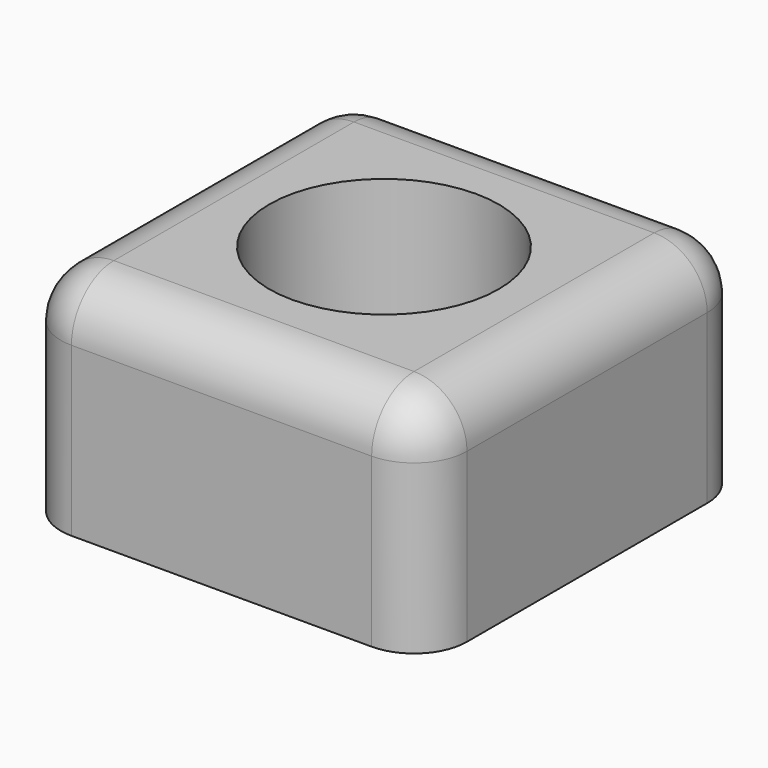
from build123d import *

# Parameters (mm, degrees)
F0_W         = 46
F0_H         = 46
F1_DEPTH     = 25
F3_DEPTH     = 15
F4_R         = 6
F5_T1_DEPTH  = 34
F5_S5_W      = 6
F5_S5_H      = 6
F5_T6_DEPTH  = 6
F5_S11_W     = 6
F5_S11_H     = 6
F5_T12_DEPTH = 6
F5_S17_W     = 6
F5_S17_H     = 6
F5_T18_DEPTH = 6
F5_S23_W     = 6
F5_S23_H     = 6
F5_T24_DEPTH = 6


# Not quite as in the source:
# - a fillet or chamfer that OpenCascade refuses, or shapes differently, is made with other operations: its cross-section is extruded or revolved along the edge and cut away or added


with BuildPart() as f1:
    # F0 (on Top) → F1 (new body)
    with BuildSketch(Plane.XY):
        with Locations((-23, 23)):
            Rectangle(F0_W, F0_H)
    extrude(amount=F1_DEPTH)

    # F2 (on face) → F3 (cut)
    with BuildSketch(Plane.XY.offset(25)):
        with BuildLine():
            ThreePointArc((-10, 23), (-32.1923881554, 32.1923881554), (-23, 10))
            ThreePointArc((-23, 10), (-13.8076118446, 13.8076118446), (-10, 23))
        make_face()
    extrude(amount=-F3_DEPTH, mode=Mode.SUBTRACT)

    # F4
    f4_edges = [f1.edges().sort_by_distance(p)[0] for p in [
        (-23, 0, 25),
        (-46, 23, 25),
        (0, 23, 25),
        (-23, 46, 25),
    ]]
    fillet(f4_edges, radius=F4_R)

    # F5: fillet of radius 6 on 4 edges, made by hand

    # F5_s2 → F5_t1 (cut)
    with BuildSketch(Plane.XY.offset(-15)):
        with BuildLine():
            ThreePointArc((-40, 0), (-44.2426406871, 1.7573593129), (-46, 6))
            Line((-46, 6), (-46, 0))
            Line((-46, 0), (-40, 0))
        make_face()
        with BuildLine():
            ThreePointArc((-6, 0), (-1.7573593129, 1.7573593129), (0, 6))
            Line((0, 6), (0, 0))
            Line((0, 0), (-6, 0))
        make_face()
        with BuildLine():
            ThreePointArc((0, 40), (-1.7573593129, 44.2426406871), (-6, 46))
            Line((-6, 46), (0, 46))
            Line((0, 46), (0, 40))
        make_face()
        with BuildLine():
            ThreePointArc((-46, 40), (-44.2426406871, 44.2426406871), (-40, 46))
            Line((-40, 46), (-46, 46))
            Line((-46, 46), (-46, 40))
        make_face()
    extrude(amount=F5_T1_DEPTH, mode=Mode.SUBTRACT)


with BuildPart() as f5_tool4:
    # F5_s5 → F5_t6 (new body)
    with BuildSketch(Plane.YZ.offset(-40)):
        with Locations((43, 22)):
            Rectangle(F5_S5_W, F5_S5_H)
    extrude(amount=-F5_T6_DEPTH)

    # F5_s7 → F5_t8 (revolve, cut)
    with BuildSketch(Plane(origin=(-40, 40, 19), x_dir=(0, -0.7071067812, -0.7071067812), z_dir=(0, 0.7071067812, -0.7071067812))):
        with BuildLine():
            ThreePointArc((0, -6), (6, 0), (0, 6))
            Line((0, 6), (0, -6))
        make_face()
    revolve(axis=Axis((-40, 40, 19), (-1, 0, 0)), mode=Mode.SUBTRACT)


with BuildPart() as f1_1:
    add(f1.part)

    # F5_t3: cut F5_tool4
    add(f5_tool4.part, mode=Mode.SUBTRACT)


with BuildPart() as f5_tool10:
    # F5_s11 → F5_t12 (new body)
    with BuildSketch(Plane.YZ.offset(-6)):
        with Locations((43, 22)):
            Rectangle(F5_S11_W, F5_S11_H)
    extrude(amount=F5_T12_DEPTH)

    # F5_s13 → F5_t14 (revolve, cut)
    with BuildSketch(Plane(origin=(-6, 40, 19), x_dir=(0, -0.7071067812, -0.7071067812), z_dir=(0, -0.7071067812, 0.7071067812))):
        with BuildLine():
            ThreePointArc((0, -6), (6, 0), (0, 6))
            Line((0, 6), (0, -6))
        make_face()
    revolve(axis=Axis((-6, 40, 19), (1, 0, 0)), mode=Mode.SUBTRACT)


with BuildPart() as f1_2:
    add(f1_1.part)

    # F5_t9: cut F5_tool10
    add(f5_tool10.part, mode=Mode.SUBTRACT)


with BuildPart() as f5_tool16:
    # F5_s17 → F5_t18 (new body)
    with BuildSketch(Plane.XZ.offset(-6)):
        with Locations((-3, 22)):
            Rectangle(F5_S17_W, F5_S17_H)
    extrude(amount=F5_T18_DEPTH)

    # F5_s19 → F5_t20 (revolve, cut)
    with BuildSketch(Plane(origin=(-6, 6, 19), x_dir=(-0.7071067812, 0, -0.7071067812), z_dir=(-0.7071067812, 0, 0.7071067812))):
        with BuildLine():
            ThreePointArc((0, -6), (6, 0), (0, 6))
            Line((0, 6), (0, -6))
        make_face()
    revolve(axis=Axis((-6, 6, 19), (0, -1, 0)), mode=Mode.SUBTRACT)


with BuildPart() as f1_3:
    add(f1_2.part)

    # F5_t15: cut F5_tool16
    add(f5_tool16.part, mode=Mode.SUBTRACT)


with BuildPart() as f5_tool22:
    # F5_s23 → F5_t24 (new body)
    with BuildSketch(Plane.XZ.offset(-6)):
        with Locations((-43, 22)):
            Rectangle(F5_S23_W, F5_S23_H)
    extrude(amount=F5_T24_DEPTH)

    # F5_s25 → F5_t26 (revolve, cut)
    with BuildSketch(Plane(origin=(-40, 6, 19), x_dir=(0.7071067812, 0, -0.7071067812), z_dir=(-0.7071067812, 0, -0.7071067812))):
        with BuildLine():
            ThreePointArc((0, -6), (6, 0), (0, 6))
            Line((0, 6), (0, -6))
        make_face()
    revolve(axis=Axis((-40, 6, 19), (0, -1, 0)), mode=Mode.SUBTRACT)


with BuildPart() as f1_4:
    add(f1_3.part)

    # F5_t21: cut F5_tool22
    add(f5_tool22.part, mode=Mode.SUBTRACT)


solid = f1_4.part
